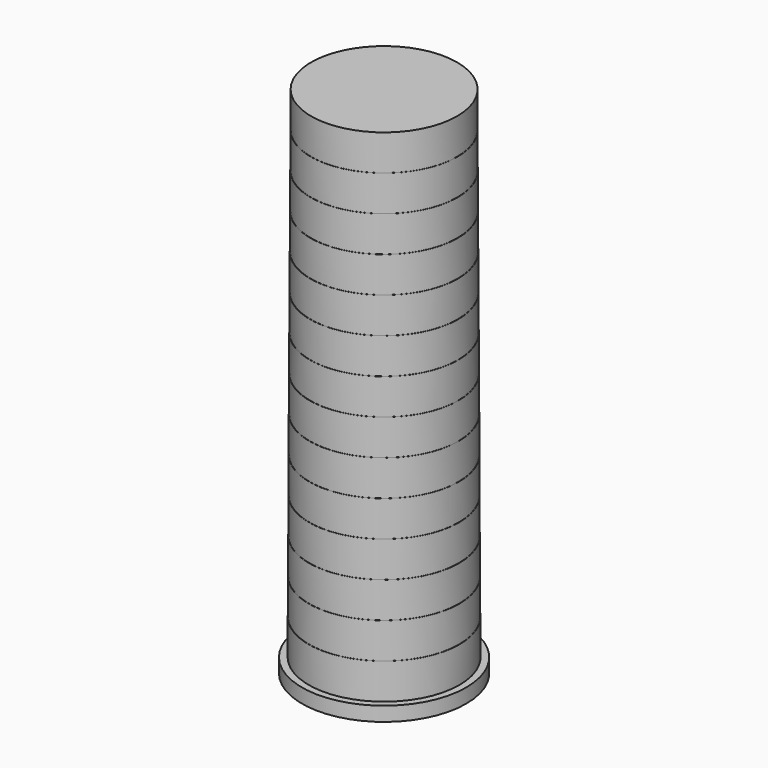
from build123d import *

# Parameters (mm, degrees)
F0_R      = 21.1
F1_DEPTH  = 10
F2_R      = 21.05
F3_DEPTH  = 10
F4_R      = 21
F5_DEPTH  = 10
F6_R      = 20.95
F7_DEPTH  = 10
F8_R      = 23
F8_R_2    = 21.1
F9_DEPTH  = 4
F10_R     = 20.9
F11_DEPTH = 10
F12_R     = 20.85
F13_DEPTH = 10
F14_R     = 20.8
F15_DEPTH = 10
F16_R     = 20.75
F17_DEPTH = 10
F18_R     = 20.7
F19_DEPTH = 10
F20_R     = 20.65
F21_DEPTH = 10
F22_R     = 20.6
F23_DEPTH = 10
F24_R     = 20.55
F25_DEPTH = 10
F26_R     = 20.5
F27_DEPTH = 10
F28_R     = 20.45
F29_DEPTH = 10


with BuildPart() as f1:
    # F0 (on Top) → F1 (new body)
    with BuildSketch(Plane.XY):
        Circle(F0_R)
    extrude(amount=F1_DEPTH)

    # F2 (on face) → F3 (join)
    with BuildSketch(Plane.XY.offset(10)):
        Circle(F2_R)
    extrude(amount=F3_DEPTH)

    # F4 (on face) → F5 (join)
    with BuildSketch(Plane.XY.offset(20)):
        Circle(F4_R)
    extrude(amount=F5_DEPTH)

    # F6 (on face) → F7 (join)
    with BuildSketch(Plane.XY.offset(30)):
        Circle(F6_R)
    extrude(amount=F7_DEPTH)

    # F8 (on face) → F9 (join)
    with BuildSketch(Plane(origin=(0, 0, 0), x_dir=(1, 0, 0), z_dir=(0, 0, -1))):
        Circle(F8_R)
        Circle(F8_R_2, mode=Mode.SUBTRACT)
        Circle(F8_R_2)
    extrude(amount=F9_DEPTH)

    # F10 (on face) → F11 (join)
    with BuildSketch(Plane.XY.offset(40)):
        Circle(F10_R)
    extrude(amount=F11_DEPTH)

    # F12 (on face) → F13 (join)
    with BuildSketch(Plane.XY.offset(50)):
        Circle(F12_R)
    extrude(amount=F13_DEPTH)

    # F14 (on face) → F15 (join)
    with BuildSketch(Plane.XY.offset(60)):
        Circle(F14_R)
    extrude(amount=F15_DEPTH)

    # F16 (on face) → F17 (join)
    with BuildSketch(Plane.XY.offset(70)):
        Circle(F16_R)
    extrude(amount=F17_DEPTH)

    # F18 (on face) → F19 (join)
    with BuildSketch(Plane.XY.offset(80)):
        Circle(F18_R)
    extrude(amount=F19_DEPTH)

    # F20 (on face) → F21 (join)
    with BuildSketch(Plane.XY.offset(90)):
        Circle(F20_R)
    extrude(amount=F21_DEPTH)

    # F22 (on face) → F23 (join)
    with BuildSketch(Plane.XY.offset(100)):
        Circle(F22_R)
    extrude(amount=F23_DEPTH)

    # F24 (on face) → F25 (join)
    with BuildSketch(Plane.XY.offset(110)):
        Circle(F24_R)
    extrude(amount=F25_DEPTH)

    # F26 (on face) → F27 (join)
    with BuildSketch(Plane.XY.offset(120)):
        Circle(F26_R)
    extrude(amount=F27_DEPTH)

    # F28 (on face) → F29 (join)
    with BuildSketch(Plane.XY.offset(130)):
        Circle(F28_R)
    extrude(amount=F29_DEPTH)


solid = f1.part
